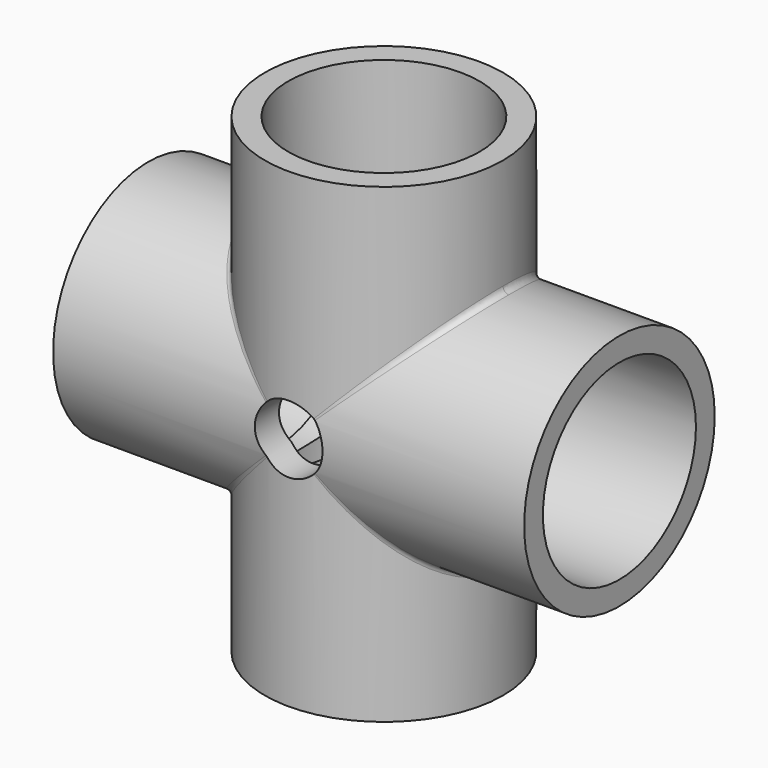
from build123d import *

# Parameters (mm, degrees)
F0_R            = 16.764
F0_R_2          = 12.5095
F1_DEPTH        = 33.147
F2_R            = 16.764
F2_R_2          = 12.5095
F3_DEPTH        = 33.147
F4_DEPTH        = 33.1480001
F4_DEPTH_BACK   = 33.1480001
F5_DEPTH        = 33.1480001
F5_DEPTH_BACK   = 33.1480001
F7_R            = 13.462
F8_DEPTH        = 18.288
F8_COPIES_COUNT = 4
F9_R            = 0.8128
F10_R           = 4.7625
F11_DEPTH       = 16.7650001
F11_DEPTH_BACK  = 16.7650001


# Not quite as in the source:
# - a pattern or mirror of a feature is missing from the dataset's text; its kind, count and spacing are read off the source's solid


with BuildPart() as f1:
    # F0 (on Right) → F1 (new body, symmetric)
    with BuildSketch(Plane.YZ):
        Circle(F0_R)
        Circle(F0_R_2, mode=Mode.SUBTRACT)
    extrude(amount=F1_DEPTH, both=True)

    # F2 (on Top) → F3 (join, symmetric)
    with BuildSketch(Plane.XY):
        Circle(F2_R)
        Circle(F2_R_2, mode=Mode.SUBTRACT)
    extrude(amount=F3_DEPTH, both=True)

    # F0 (on Right) → F4 (cut, two sides)
    with BuildSketch(Plane.YZ) as f4_sk:
        Circle(F0_R_2)
    extrude(amount=-F4_DEPTH, mode=Mode.SUBTRACT)
    extrude(f4_sk.sketch, amount=F4_DEPTH_BACK, mode=Mode.SUBTRACT)

    # F2 (on Top) → F5 (cut, two sides)
    with BuildSketch(Plane.XY) as f5_sk:
        Circle(F2_R_2)
    extrude(amount=-F5_DEPTH, mode=Mode.SUBTRACT)
    extrude(f5_sk.sketch, amount=F5_DEPTH_BACK, mode=Mode.SUBTRACT)

    # F7 (on face) → F8 (cut)
    with BuildSketch(Plane.YZ.offset(33.147)):
        Circle(F7_R)
    f8 = extrude(amount=-F8_DEPTH, mode=Mode.SUBTRACT)

    # F8_copies: F8 ×4 about axis
    f8_copies_axis = Axis((0, 0, 0), (0, 1, 0))
    for i in range(1, F8_COPIES_COUNT):
        add(f8.rotate(f8_copies_axis, i * 360 / F8_COPIES_COUNT), mode=Mode.SUBTRACT)

    # F9
    f9_edges = [f1.edges().sort_by_distance(p)[0] for p in [
        (-16.764, -1.8e-05, 16.764),
        (-16.764, 1.8e-05, -16.764),
        (10.830364, 12.795894, -10.830364),
        (10.830364, -12.795894, -10.830364),
        (10.830364, -12.795894, 10.830364),
        (10.830364, 12.795894, 10.830364),
    ]]
    fillet(f9_edges, radius=F9_R)

    # F10 (on Front) → F11 (cut, two sides)
    with BuildSketch(Plane.XZ) as f11_sk:
        Circle(F10_R)
    extrude(amount=-F11_DEPTH, mode=Mode.SUBTRACT)
    extrude(f11_sk.sketch, amount=F11_DEPTH_BACK, mode=Mode.SUBTRACT)


solid = f1.part
